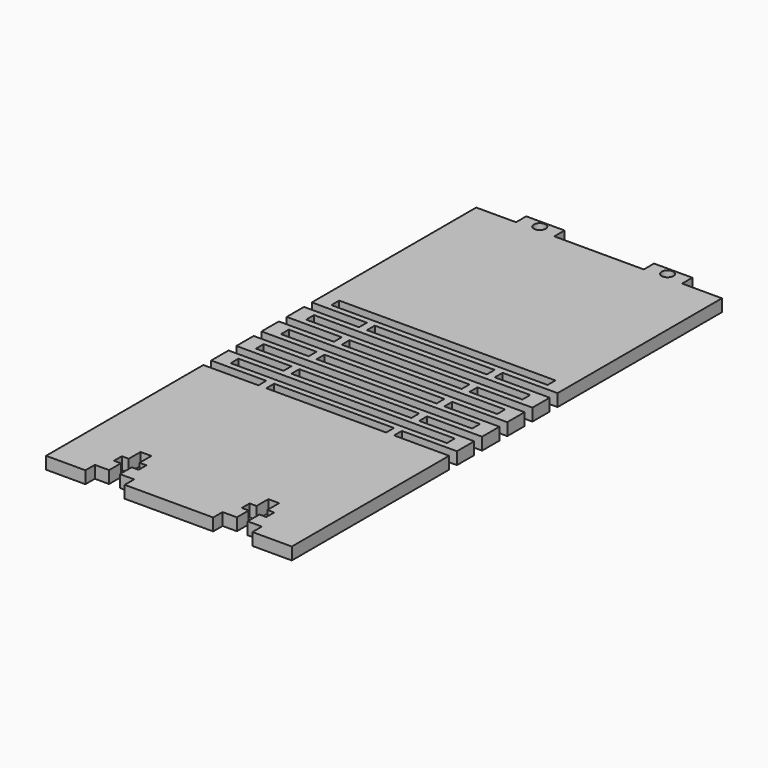
from build123d import *

# Parameters (mm, degrees)
F0_W     = 30.988
F0_H     = 2.54
F0_W_2   = 55.88
F0_R     = 1.524
F1_DEPTH = 3.175


# Not quite as in the source:
# - a length typed as a fraction of an inch, garbled in the dataset ("3 / 203.2 mm" for 3/8 in), is restored
# - a feature names something its author has since deleted; it is built from what else it names


with BuildPart() as f1:
    # F0 (on Top) → F1 (new body)
    with BuildSketch(Plane.XY):
        Polygon((21.59, -64.4452290503), (31.75, -64.4452290503), (31.75, -13.6452290503), (17.526, -13.6452290503), (17.526, -11.1052290503), (31.75, -11.1052290503), (31.75, -5.5172290503), (17.526, -5.5172290503), (17.526, -2.9772290503), (31.75, -2.9772290503), (31.75, 2.6107709497), (17.526, 2.6107709497), (17.526, 5.1507709497), (31.75, 5.1507709497), (31.75, 10.7387709497), (17.526, 10.7387709497), (17.526, 13.2787709497), (31.75, 13.2787709497), (31.75, 18.8667709497), (17.526, 18.8667709497), (17.526, 21.4067709497), (31.75, 21.4067709497), (31.75, 26.9947709497), (-31.75, 26.9947709497), (-31.75, 21.4067709497), (-17.526, 21.4067709497), (-17.526, 18.8667709497), (-31.75, 18.8667709497), (-31.75, 13.2787709497), (-17.526, 13.2787709497), (-17.526, 10.7387709497), (-31.75, 10.7387709497), (-31.75, 5.1507709497), (-17.526, 5.1507709497), (-17.526, 2.6107709497), (-31.75, 2.6107709497), (-31.75, -2.9772290503), (-17.526, -2.9772290503), (-17.526, -5.5172290503), (-31.75, -5.5172290503), (-31.75, -11.1052290503), (-17.526, -11.1052290503), (-17.526, -13.6452290503), (-31.75, -13.6452290503), (-31.75, -64.4452290503), (-21.59, -64.4452290503), (-21.59, -61.3972290503), (-17.907, -61.3972290503), (-17.907, -57.5872290503), (-19.685, -57.5872290503), (-19.685, -55.0472290503), (-17.907, -55.0472290503), (-17.907, -51.2372290503), (-15.113, -51.2372290503), (-15.113, -55.0472290503), (-13.335, -55.0472290503), (-13.335, -57.5872290503), (-15.113, -57.5872290503), (-15.113, -61.3972290503), (-11.43, -61.3972290503), (-11.43, -64.4452290503), (11.43, -64.4452290503), (11.43, -61.3972290503), (15.113, -61.3972290503), (15.113, -57.5872290503), (13.335, -57.5872290503), (13.335, -55.0472290503), (15.113, -55.0472290503), (15.113, -51.2372290503), (17.907, -51.2372290503), (17.907, -55.0472290503), (19.685, -55.0472290503), (19.685, -57.5872290503), (17.907, -57.5872290503), (17.907, -61.3972290503), (21.59, -61.3972290503), align=None)
        with Locations((0, -12.3752290503)):
            Rectangle(F0_W, F0_H, mode=Mode.SUBTRACT)
        with Locations((0, -8.3112290503)):
            Rectangle(F0_W_2, F0_H, mode=Mode.SUBTRACT)
        with Locations((0, -4.2472290503)):
            Rectangle(F0_W, F0_H, mode=Mode.SUBTRACT)
        with Locations((0, -0.1832290503)):
            Rectangle(F0_W_2, F0_H, mode=Mode.SUBTRACT)
        with Locations((0, 3.8807709497)):
            Rectangle(F0_W, F0_H, mode=Mode.SUBTRACT)
        with Locations((0, 7.9447709497)):
            Rectangle(F0_W_2, F0_H, mode=Mode.SUBTRACT)
        with Locations((0, 12.0087709497)):
            Rectangle(F0_W, F0_H, mode=Mode.SUBTRACT)
        with Locations((0, 16.0727709497)):
            Rectangle(F0_W_2, F0_H, mode=Mode.SUBTRACT)
        with Locations((0, 20.1367709497)):
            Rectangle(F0_W, F0_H, mode=Mode.SUBTRACT)
        with Locations((0, 24.2007709497)):
            Rectangle(F0_W_2, F0_H, mode=Mode.SUBTRACT)
        Polygon((-31.75, 26.9947709497), (31.75, 26.9947709497), (31.75, 74.4927709497), (21.463, 74.4927709497), (21.463, 77.7947709497), (11.557, 77.7947709497), (11.557, 74.4927709497), (-11.557, 74.4927709497), (-11.557, 77.7947709497), (-21.463, 77.7947709497), (-21.463, 74.4927709497), (-31.75, 74.4927709497), align=None)
        with Locations((-16.51, 75.9786709497)):
            Circle(F0_R, mode=Mode.SUBTRACT)
        with Locations((16.51, 75.9786709497)):
            Circle(F0_R, mode=Mode.SUBTRACT)
    extrude(amount=F1_DEPTH)


solid = f1.part
